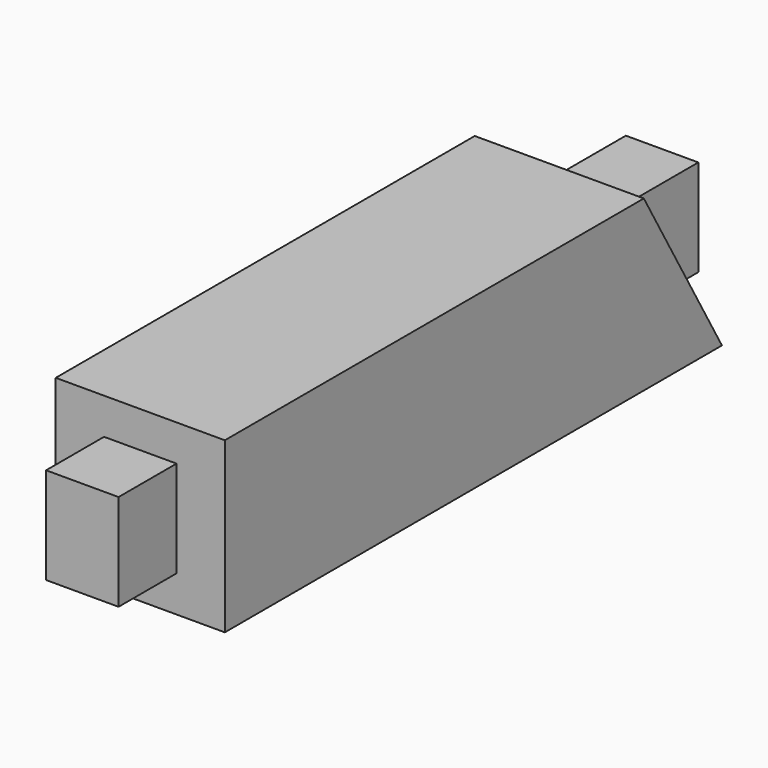
from build123d import *

# Parameters (mm, degrees)
F0_W     = 381
F0_H     = 88.9
F1_DEPTH = 44.45
F4_W     = 88.9
F4_H     = 88.9
F4_W_2   = 38.1
F4_H_2   = 50.8
F5_REACH = 193.287585695
F6_W     = 88.9
F6_H     = 88.9
F6_W_2   = 38.1
F6_H_2   = 50.8
F7_DEPTH = 38.1


with BuildPart() as f1:
    # F0 (on Right) → F1 (new body, symmetric)
    with BuildSketch(Plane.YZ):
        Rectangle(F0_W, F0_H)
    extrude(amount=F1_DEPTH, both=True)

    f5_end = Plane(origin=(0, 111.4494145991, 64.3453495198), x_dir=(0, -0.5, 0.8660254038), z_dir=(0, 0.8660254038, 0.5))
    # F4 (on face) → F5 (cut, up to a plane its end follows)
    with BuildSketch(Plane(origin=(0, 190.5, 0), x_dir=(-1, 0, 0), z_dir=(0, 1, 0))):
        Rectangle(F4_W, F4_H)
        Rectangle(F4_W_2, F4_H_2, mode=Mode.SUBTRACT)
    f5_long = extrude(amount=-F5_REACH, mode=Mode.PRIVATE)
    add(split(f5_long, bisect_by=f5_end, keep=Keep.TOP, mode=Mode.PRIVATE), mode=Mode.SUBTRACT)

    # F6 (on face) → F7 (cut)
    with BuildSketch(Plane.XZ.offset(190.5)):
        Rectangle(F6_W, F6_H)
        Rectangle(F6_W_2, F6_H_2, mode=Mode.SUBTRACT)
    extrude(amount=-F7_DEPTH, mode=Mode.SUBTRACT)


solid = f1.part
